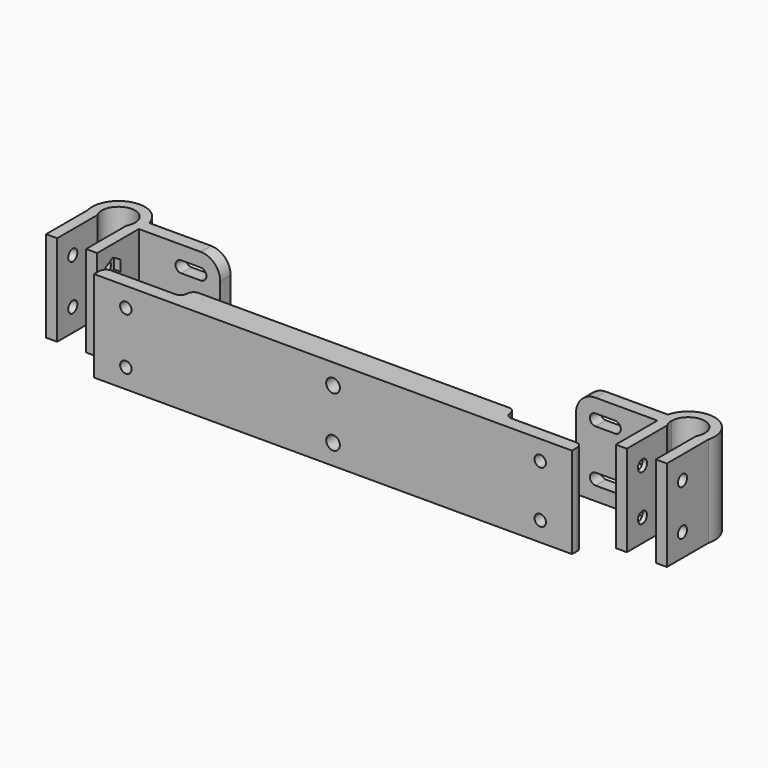
from build123d import *

# Parameters (mm, degrees)
F1_DEPTH  = 28
F2_R      = 1.75
F4_DEPTH  = 2
F5_DEPTH  = 25
F6_DEPTH  = 25
F7_R      = 6
F10_W     = 23.75
F10_H     = 28
F10_R     = 1.75
F11_DEPTH = 4
F10_W_2   = 49.6507962187
F12_DEPTH = 8
F13_R     = 1.99999
F15_R     = 2.1
F16_DEPTH = 2
F17_DEPTH = 25


# Not quite as in the source:
# - a fillet or chamfer is up to 0.001 mm smaller than in the source, because OpenCascade refuses the exact size


with BuildPart() as f1:
    # F0 (on Top) → F1 (new body)
    with BuildSketch(Plane.XY):
        with BuildLine():
            Line((-91.9452221542, -18), (-91.9452221542, -6.7712628069))
            ThreePointArc((-91.9452221542, -6.7712628069), (-94.0938960004, -4.7043103146), (-95.3492037813, -2))
            Line((-95.3492037813, -2), (-95.3492037813, -18))
            Line((-95.3492037813, -18), (-91.9452221542, -18))
        make_face()
        with BuildLine():
            Line((-91.9452221542, -6.7712628069), (-91.9452221542, -2.5))
            ThreePointArc((-91.9452221542, -2.5), (-92.0751873258, -2.2533665778), (-92.1914816423, -2))
            Line((-92.1914816423, -2), (-95.3492037813, -2))
            ThreePointArc((-95.3492037813, -2), (-94.0938960004, -4.7043103146), (-91.9452221542, -6.7712628069))
        make_face()
        with BuildLine():
            Line((-95.3492037813, -2), (-92.1914816423, -2))
            ThreePointArc((-92.1914816423, -2), (-88.5206477415, 4.9968268119), (-82.4, 0))
            ThreePointArc((-82.4, 0), (-82.5031731881, -1.0206477415), (-82.8085183577, -2))
            Line((-82.8085183577, -2), (-79.6507962187, -2))
            Line((-79.6507962187, -2), (-79.6507962187, 2))
            ThreePointArc((-79.6507962187, 2), (-89.5, 7.8492037813), (-95.3492037813, -2))
        make_face()
        with BuildLine():
            ThreePointArc((-79.6507962187, -2), (-80.9061039996, -4.7043103146), (-83.0547778458, -6.7712628069))
            Line((-83.0547778458, -6.7712628069), (-83.0547778458, -18))
            Line((-83.0547778458, -18), (-79.6507962187, -18))
            Line((-79.6507962187, -18), (-79.6507962187, -2))
        make_face()
        with BuildLine():
            ThreePointArc((-82.8085183577, -2), (-82.9248126742, -2.2533665778), (-83.0547778458, -2.5))
            Line((-83.0547778458, -2.5), (-83.0547778458, -6.7712628069))
            ThreePointArc((-83.0547778458, -6.7712628069), (-80.9061039996, -4.7043103146), (-79.6507962187, -2))
            Line((-79.6507962187, -2), (-82.8085183577, -2))
        make_face()
        with BuildLine():
            ThreePointArc((-79.4, 0), (-79.4629436163, -1.0078316753), (-79.6507962187, -2))
            Line((-79.6507962187, -2), (-54.6507962187, -2))
            Line((-54.6507962187, -2), (-54.6507962187, 2))
            Line((-54.6507962187, 2), (-79.6507962187, 2))
            ThreePointArc((-79.6507962187, 2), (-79.4629436163, 1.0078316753), (-79.4, 0))
        make_face()
        with BuildLine():
            Line((-79.6507962187, 2), (-79.6507962187, -2))
            ThreePointArc((-79.6507962187, -2), (-79.4629436163, -1.0078316753), (-79.4, 0))
            ThreePointArc((-79.4, 0), (-79.4629436163, 1.0078316753), (-79.6507962187, 2))
        make_face()
    extrude(amount=F1_DEPTH)

    # F2 (on face) → F4 (cut)
    with BuildSketch(Plane.YZ.offset(-79.6507962187)):
        Polygon((-14.9, 19.3256842194), (-12, 17.6513684387), (-9.1, 19.3256842194), (-9.1, 22.6743157806), (-12, 24.3486315613), (-14.9, 22.6743157806), align=None)
        with Locations((-12, 21)):
            Circle(F2_R, mode=Mode.SUBTRACT)
        Polygon((-9.1, 8.6743157806), (-12, 10.3486315613), (-14.9, 8.6743157806), (-14.9, 5.3256842194), (-12, 3.6513684387), (-9.1, 5.3256842194), align=None)
        with Locations((-12, 7)):
            Circle(F2_R, mode=Mode.SUBTRACT)
    extrude(amount=-F4_DEPTH, mode=Mode.SUBTRACT)

    # F5 (cut): faces of the model
    f5_faces = [f1.faces().sort_by_distance(p)[0] for p in [
        (-79.6507962187, -12, 21),
        (-79.6507962187, -12, 7),
    ]]
    extrude(f5_faces, amount=-F5_DEPTH, mode=Mode.SUBTRACT)

    # F3 (on face) → F6 (cut)
    with BuildSketch(Plane(origin=(0, 2, 0), x_dir=(-1, 0, 0), z_dir=(0, 1, 0))):
        with BuildLine():
            ThreePointArc((60.6507962187, 23.75), (58.9007962187, 22), (60.6507962187, 20.25))
            Line((60.6507962187, 20.25), (66.6507962187, 20.25))
            ThreePointArc((66.6507962187, 20.25), (68.4007962187, 22), (66.6507962187, 23.75))
            Line((66.6507962187, 23.75), (60.6507962187, 23.75))
        make_face()
        with BuildLine():
            ThreePointArc((60.6507962187, 7.75), (58.9007962187, 6), (60.6507962187, 4.25))
            Line((60.6507962187, 4.25), (66.6507962187, 4.25))
            ThreePointArc((66.6507962187, 4.25), (68.4007962187, 6), (66.6507962187, 7.75))
            Line((66.6507962187, 7.75), (60.6507962187, 7.75))
        make_face()
    extrude(amount=-F6_DEPTH, mode=Mode.SUBTRACT)

    # F7
    f7_edges = [f1.edges().sort_by_distance(p)[0] for p in [
        (-54.650796, 0, 28),
    ]]
    fillet(f7_edges, radius=F7_R)


with BuildPart() as f8_1:
    # F8: instance of F1
    add(f1.part.mirror(Plane.YZ))


with BuildPart() as f11:
    # F10 (on offset) → F11 (new body)
    with BuildSketch(Plane.XZ.offset(27)):
        with Locations((-61.5257962187, 14)):
            Rectangle(F10_W, F10_H)
        with Locations((-63.6507962187, 6)):
            Circle(F10_R, mode=Mode.SUBTRACT)
        with Locations((-63.6507962187, 22)):
            Circle(F10_R, mode=Mode.SUBTRACT)
    extrude(amount=-F11_DEPTH)

    # F10 (on offset) → F12 (join)
    with BuildSketch(Plane.XZ.offset(27)):
        with Locations((-24.8253981094, 14)):
            Rectangle(F10_W_2, F10_H)
    extrude(amount=-F12_DEPTH)

    # F13 (radius 2 in the source; OpenCascade refuses exactly that, so slightly less here)
    f13_edges = [f11.edges().sort_by_distance(p)[0] for p in [
        (-73.400796, -23, 14),
        (-49.650796, -19, 14),
        (-49.650796, -23, 14),
    ]]
    fillet(f13_edges, radius=F13_R)

    # F14: F11 across plane


with BuildPart() as f11_1:
    add(f11.part)
    add(f11.part.mirror(Plane.YZ))

    # F15 (on face) → F16 (cut)
    with BuildSketch(Plane(origin=(0, -19, 0), x_dir=(-1, 0, 0), z_dir=(0, 1, 0))):
        Polygon((3.65, 8.3573284825), (0, 10.4646569651), (-3.65, 8.3573284825), (-3.65, 4.1426715175), (0, 2.0353430349), (3.65, 4.1426715175), align=None)
        with Locations((0, 6.25)):
            Circle(F15_R, mode=Mode.SUBTRACT)
        Polygon((-3.65, 19.6426715175), (0, 17.5353430349), (3.65, 19.6426715175), (3.65, 23.8573284825), (0, 25.9646569651), (-3.65, 23.8573284825), align=None)
        with Locations((0, 21.75)):
            Circle(F15_R, mode=Mode.SUBTRACT)
    extrude(amount=-F16_DEPTH, mode=Mode.SUBTRACT)

    # F17 (cut): faces of the model
    f17_faces = [f11_1.faces().sort_by_distance(p)[0] for p in [
        (0, -19, 21.75),
        (0, -19, 6.25),
    ]]
    extrude(f17_faces, amount=-F17_DEPTH, mode=Mode.SUBTRACT)


solid = Compound([f1.part, f8_1.part, f11_1.part])
